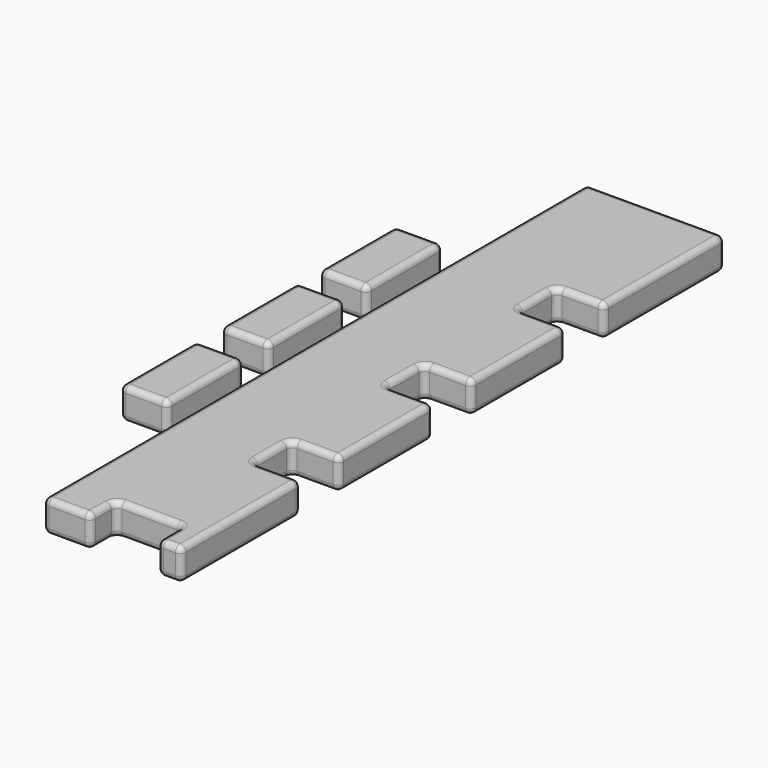
from build123d import *

# Parameters (mm, degrees)
F1_DEPTH  = 26.8
F0_W      = 40.5
F0_H      = 81
F2_F1_R   = 5
F2_F2_R   = 5
F2_2_F1_R = 5
F2_2_F2_R = 5
F2_2_F3_R = 5
F2_2_F4_R = 5
F2_2_F5_R = 5
F2_3_F1_R = 5
F2_3_F2_R = 5
F2_3_F3_R = 5
F2_3_F4_R = 5
F2_3_F5_R = 5
F2_4_F1_R = 5
F2_4_F2_R = 5
F2_4_F3_R = 5
F2_4_F4_R = 5
F2_4_F5_R = 5


with BuildPart() as f1:
    # F0 (on Top) → F1 (new body)
    with BuildSketch(Plane.XY):
        Polygon((-13.4848476946, 483.5782089114), (-94.4848476946, 483.5782089114), (-94.4848476946, -66.4217910886), (-94.4848476946, -93.2217910886), (-53.9848476946, -93.2217910886), (-53.9848476946, -66.4217910886), (2.7238028377, -66.4217910886), (2.7238028377, -93.2217910886), (22.9238028377, -93.2217910886), (22.9238028377, -66.4217910886), (22.9238028377, 33.5782089114), (-17.5761971623, 33.5782089114), (-17.5761971623, 74.0782089114), (22.9238028377, 74.0782089114), (22.9238028377, 174.0782089114), (-17.5761971623, 174.0782089114), (-17.5761971623, 214.5782089114), (22.9238028377, 214.5782089114), (22.9238028377, 314.5782089114), (-17.5761971623, 314.5782089114), (-17.5761971623, 355.0782089114), (22.9238028377, 355.0782089114), (22.9238028377, 483.5782089114), align=None)
    extrude(amount=F1_DEPTH)

    # F2: fillet of radius 5 on 54 edges, made by hand

    # F2_f1
    f2_f1_edges = [f1.edges().sort_by_distance(p)[0] for p in [
        (-17.5761971623, 314.5782089114, 13.4),
        (-17.5761971623, 355.0782089114, 13.4),
        (-17.5761971623, 174.0782089114, 13.4),
        (-17.5761971623, 214.5782089114, 13.4),
        (-17.5761971623, 33.5782089114, 13.4),
        (-17.5761971623, 74.0782089114, 13.4),
        (-53.9848476946, -66.4217910886, 13.4),
        (2.7238028377, -66.4217910886, 13.4),
    ]]
    fillet(f2_f1_edges, radius=F2_F1_R)

    # F2_f2
    f2_f2_edges = [f1.edges().sort_by_distance(p)[0] for p in [
        (22.9238028377, 214.5782089114, 13.4),
        (22.9238028377, 314.5782089114, 13.4),
        (22.9238028377, 264.5782089114, 0),
        (22.9238028377, 264.5782089114, 26.8),
        (22.9238028377, 355.0782089114, 13.4),
        (22.9238028377, 483.5782089114, 13.4),
        (22.9238028377, 419.3282089114, 0),
        (22.9238028377, 419.3282089114, 26.8),
        (-17.5761971623, 334.8282089114, 0),
        (-17.5761971623, 334.8282089114, 26.8),
        (-17.5761971623, 194.3282089114, 0),
        (-17.5761971623, 194.3282089114, 26.8),
        (22.9238028377, 74.0782089114, 13.4),
        (22.9238028377, 174.0782089114, 13.4),
        (22.9238028377, 124.0782089114, 0),
        (22.9238028377, 124.0782089114, 26.8),
        (-17.5761971623, 53.8282089114, 0),
        (-17.5761971623, 53.8282089114, 26.8),
        (22.9238028377, -93.2217910886, 13.4),
        (22.9238028377, -29.8217910886, 26.8),
        (22.9238028377, 33.5782089114, 13.4),
        (22.9238028377, -29.8217910886, 0),
        (-25.6305224285, -66.4217910886, 0),
        (-25.6305224285, -66.4217910886, 26.8),
        (2.7238028377, -93.2217910886, 13.4),
        (12.8238028377, -93.2217910886, 0),
        (12.8238028377, -93.2217910886, 26.8),
        (-94.4848476946, -93.2217910886, 13.4),
        (-53.9848476946, -93.2217910886, 13.4),
        (-74.2348476946, -93.2217910886, 0),
        (-74.2348476946, -93.2217910886, 26.8),
        (-94.4848476946, 483.5782089114, 13.4),
        (-35.7805224285, 483.5782089114, 0),
        (-35.7805224285, 483.5782089114, 26.8),
        (-94.4848476946, 195.1782089114, 26.8),
        (-94.4848476946, 195.1782089114, 0),
        (5.1738028377, 174.0782089114, 0),
        (5.1738028377, 74.0782089114, 26.8),
        (5.1738028377, 33.5782089114, 0),
        (5.1738028377, 355.0782089114, 26.8),
        (5.1738028377, 314.5782089114, 0),
        (-53.9848476946, -82.3217910886, 0),
        (2.7238028377, -82.3217910886, 0),
        (5.1738028377, 74.0782089114, 0),
        (5.1738028377, 214.5782089114, 0),
        (5.1738028377, 355.0782089114, 0),
        (-16.1117310682, 353.6137428174, 0),
        (-16.1117310682, 213.1137428174, 0),
        (-16.1117310682, 72.6137428174, 0),
        (1.2593367437, -67.8862571826, 0),
        (-52.5203816006, -67.8862571826, 0),
        (-16.1117310682, 316.0426750055, 0),
        (-16.1117310682, 353.6137428174, 26.8),
        (-16.1117310682, 35.0426750055, 0),
        (-16.1117310682, 72.6137428174, 26.8),
        (-16.1117310682, 175.5426750055, 0),
        (-52.5203816006, -67.8862571826, 26.8),
        (1.2593367437, -67.8862571826, 26.8),
        (-16.1117310682, 35.0426750055, 26.8),
        (-16.1117310682, 175.5426750055, 26.8),
        (-16.1117310682, 213.1137428174, 26.8),
        (-16.1117310682, 316.0426750055, 26.8),
    ]]
    fillet(f2_f2_edges, radius=F2_F2_R)


with BuildPart() as f1b:
    # F0 (on Top) → F1, piece 2 (new body)
    with BuildSketch(Plane.XY):
        with Locations((-135.7250287533, 317.0576243401)):
            Rectangle(F0_W, F0_H)
    extrude(amount=F1_DEPTH)

    # F2#4: fillet of radius 5 on 12 edges, made by hand

    # F2_4_f1
    f2_4_f1_edges = [f1b.edges().sort_by_distance(p)[0] for p in [
        (-115.4750287533, 357.5576243401, 13.4),
    ]]
    fillet(f2_4_f1_edges, radius=F2_4_F1_R)

    # F2_4_f2
    f2_4_f2_edges = [f1b.edges().sort_by_distance(p)[0] for p in [
        (-155.9750287533, 357.5576243401, 13.4),
    ]]
    fillet(f2_4_f2_edges, radius=F2_4_F2_R)

    # F2_4_f3
    f2_4_f3_edges = [f1b.edges().sort_by_distance(p)[0] for p in [
        (-135.7250287533, 357.5576243401, 0),
    ]]
    fillet(f2_4_f3_edges, radius=F2_4_F3_R)

    # F2_4_f4
    f2_4_f4_edges = [f1b.edges().sort_by_distance(p)[0] for p in [
        (-135.7250287533, 357.5576243401, 26.8),
    ]]
    fillet(f2_4_f4_edges, radius=F2_4_F4_R)

    # F2_4_f5
    f2_4_f5_edges = [f1b.edges().sort_by_distance(p)[0] for p in [
        (-155.9750287533, 276.5576243401, 13.4),
    ]]
    fillet(f2_4_f5_edges, radius=F2_4_F5_R)


with BuildPart() as f1c:
    # F0 (on Top) → F1, piece 3 (new body)
    with BuildSketch(Plane.XY):
        with Locations((-135.7250287533, 212.9805533886)):
            Rectangle(F0_W, F0_H)
    extrude(amount=F1_DEPTH)

    # F2#3: fillet of radius 5 on 12 edges, made by hand

    # F2_3_f1
    f2_3_f1_edges = [f1c.edges().sort_by_distance(p)[0] for p in [
        (-115.4750287533, 253.4805533886, 13.4),
    ]]
    fillet(f2_3_f1_edges, radius=F2_3_F1_R)

    # F2_3_f2
    f2_3_f2_edges = [f1c.edges().sort_by_distance(p)[0] for p in [
        (-155.9750287533, 253.4805533886, 13.4),
    ]]
    fillet(f2_3_f2_edges, radius=F2_3_F2_R)

    # F2_3_f3
    f2_3_f3_edges = [f1c.edges().sort_by_distance(p)[0] for p in [
        (-135.7250287533, 253.4805533886, 0),
    ]]
    fillet(f2_3_f3_edges, radius=F2_3_F3_R)

    # F2_3_f4
    f2_3_f4_edges = [f1c.edges().sort_by_distance(p)[0] for p in [
        (-135.7250287533, 253.4805533886, 26.8),
    ]]
    fillet(f2_3_f4_edges, radius=F2_3_F4_R)

    # F2_3_f5
    f2_3_f5_edges = [f1c.edges().sort_by_distance(p)[0] for p in [
        (-155.9750287533, 172.4805533886, 13.4),
    ]]
    fillet(f2_3_f5_edges, radius=F2_3_F5_R)


with BuildPart() as f1d:
    # F0 (on Top) → F1, piece 4 (new body)
    with BuildSketch(Plane.XY):
        with Locations((-135.7250287533, 105.5818645954)):
            Rectangle(F0_W, F0_H)
    extrude(amount=F1_DEPTH)

    # F2#2: fillet of radius 5 on 12 edges, made by hand

    # F2_2_f1
    f2_2_f1_edges = [f1d.edges().sort_by_distance(p)[0] for p in [
        (-115.4750287533, 146.0818645954, 13.4),
    ]]
    fillet(f2_2_f1_edges, radius=F2_2_F1_R)

    # F2_2_f2
    f2_2_f2_edges = [f1d.edges().sort_by_distance(p)[0] for p in [
        (-155.9750287533, 146.0818645954, 13.4),
    ]]
    fillet(f2_2_f2_edges, radius=F2_2_F2_R)

    # F2_2_f3
    f2_2_f3_edges = [f1d.edges().sort_by_distance(p)[0] for p in [
        (-135.7250287533, 146.0818645954, 0),
    ]]
    fillet(f2_2_f3_edges, radius=F2_2_F3_R)

    # F2_2_f4
    f2_2_f4_edges = [f1d.edges().sort_by_distance(p)[0] for p in [
        (-135.7250287533, 146.0818645954, 26.8),
    ]]
    fillet(f2_2_f4_edges, radius=F2_2_F4_R)

    # F2_2_f5
    f2_2_f5_edges = [f1d.edges().sort_by_distance(p)[0] for p in [
        (-155.9750287533, 65.0818645954, 13.4),
    ]]
    fillet(f2_2_f5_edges, radius=F2_2_F5_R)


solid = Compound([f1.part, f1b.part, f1c.part, f1d.part])
